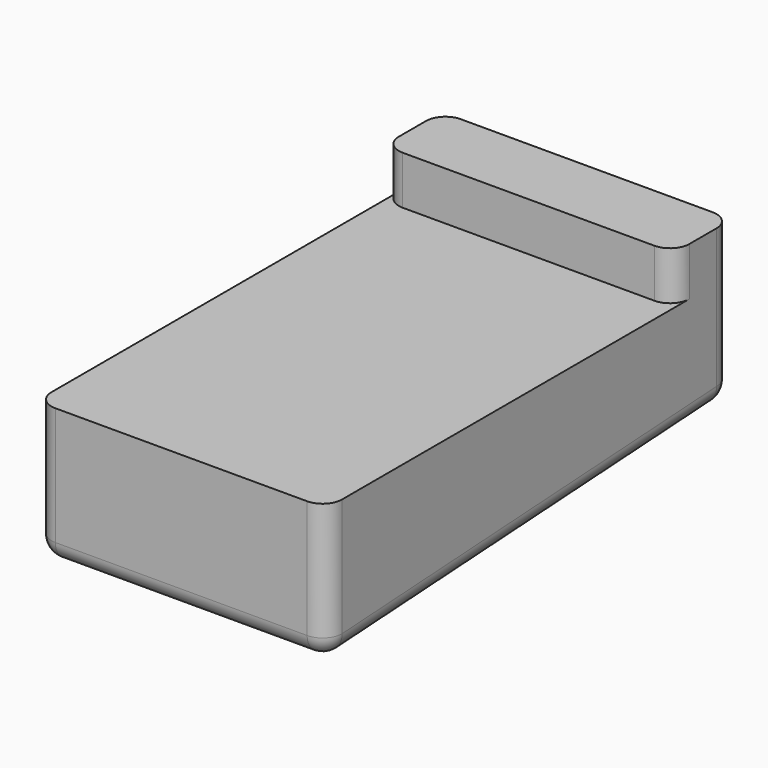
from build123d import *

# Parameters (mm, degrees)
F2_DEPTH = 76.2
F3_R     = 5.08


# Not quite as in the source:
# - a feature names something its author has since deleted; it is built from what else it names


with BuildPart() as f2:
    # F1 (on offset) → F2 (new body)
    with BuildSketch(Plane.YZ.offset(76.2)):
        Polygon((0, -41.275), (0, 0), (-19.05, 0), (-19.05, -12.7), (-132.9298521399, -12.7), (-132.9298521399, -49.0773997059), align=None)
    extrude(amount=-F2_DEPTH)

    # F3
    f3_edges = [f2.edges().sort_by_distance(p)[0] for p in [
        (38.1, 0, -41.275),
        (76.2, 0, -20.6375),
        (0, 0, -20.6375),
        (76.2, -66.464926, -45.1762),
        (0, -66.464926, -45.1762),
        (0, -19.05, -6.35),
        (76.2, -19.05, -6.35),
        (0, -132.929852, -30.8887),
        (76.2, -132.929852, -30.8887),
        (38.1, -132.929852, -49.0774),
    ]]
    fillet(f3_edges, radius=F3_R)


solid = f2.part
